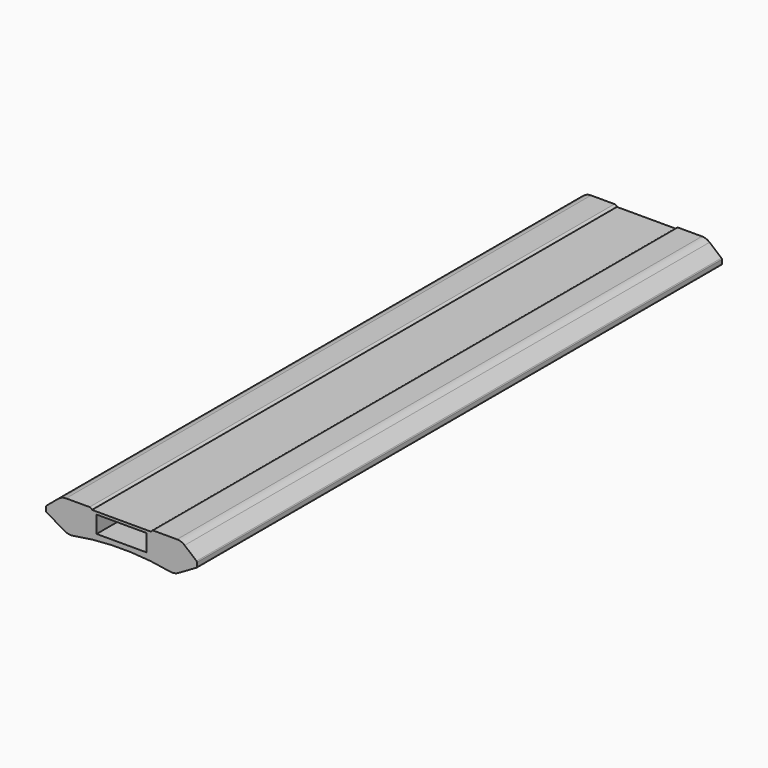
from build123d import *

# Parameters (mm, degrees)
F1_DEPTH    = 250
F2_W        = 38
F2_H        = 13
F3_DEPTH    = 250
F4_T1_DEPTH = 509.3674969976
F5_R        = 9
F6_R        = 1


# Not quite as in the source:
# - a fillet or chamfer that OpenCascade refuses, or shapes differently, is made with other operations: its cross-section is extruded or revolved along the edge and cut away or added


with BuildPart() as f1:
    # F0 (on Front) → F1 (new body, symmetric)
    with BuildSketch(Plane.XZ):
        with BuildLine():
            Line((22.5, 16.4041765079), (0, 16.4041765079))
            Line((0, 16.4041765079), (-22.5, 16.4041765079))
            Line((-22.5, 16.4041765079), (-22.5, 17.7041765079))
            Line((-22.5, 17.7041765079), (-45.5824640741, 17.7041765079))
            Line((-45.5824640741, 17.7041765079), (-57.5, 7.7041765079))
            Line((-57.5, 7.7041765079), (-57.5, 3.7041765079))
            Line((-57.5, 3.7041765079), (-40.1794919243, -6.2958234921))
            ThreePointArc((-40.1794919243, -6.2958234921), (0, -2.2182786337), (40.1794919243, -6.2958234921))
            Line((40.1794919243, -6.2958234921), (57.5, 3.7041765079))
            Line((57.5, 3.7041765079), (57.5, 7.7041765079))
            Line((57.5, 7.7041765079), (45.5824640741, 17.7041765079))
            Line((45.5824640741, 17.7041765079), (22.5, 17.7041765079))
            Line((22.5, 17.7041765079), (22.5, 16.4041765079))
        make_face()
    extrude(amount=F1_DEPTH, both=True)

    # F2 (on Front) → F3 (cut, symmetric)
    with BuildSketch(Plane.XZ):
        with Locations((0, 7.9041765079)):
            Rectangle(F2_W, F2_H)
    extrude(amount=F3_DEPTH, both=True, mode=Mode.SUBTRACT)

    # F4: fillet of radius 2 on 2 edges, made by hand

    # F4_s2 → F4_t1 (cut)
    with BuildSketch(Plane.XZ.offset(-254.6837484988)):
        with BuildLine():
            ThreePointArc((-22.5, 16.4041765079), (-23.2333239744, 17.3473441804), (-24.3734993995, 17.7041765079))
            Line((-24.3734993995, 17.7041765079), (-22.5, 17.7041765079))
            Line((-22.5, 17.7041765079), (-22.5, 16.4041765079))
        make_face()
        with BuildLine():
            ThreePointArc((24.3734993995, 17.7041765079), (23.2333239744, 17.3473441804), (22.5, 16.4041765079))
            Line((22.5, 16.4041765079), (22.5, 17.7041765079))
            Line((22.5, 17.7041765079), (24.3734993995, 17.7041765079))
        make_face()
    extrude(amount=F4_T1_DEPTH, mode=Mode.SUBTRACT)

    # F5
    f5_edges = [f1.edges().sort_by_distance(p)[0] for p in [
        (45.582464, 0, 17.704177),
        (40.179492, 0, -6.295823),
        (-40.179492, 0, -6.295823),
        (-45.582464, 0, 17.704177),
    ]]
    fillet(f5_edges, radius=F5_R)

    # F6
    f6_edges = [f1.edges().sort_by_distance(p)[0] for p in [
        (57.5, 0, 3.704177),
        (57.5, 0, 7.704177),
        (-57.5, 0, 7.704177),
        (-57.5, 0, 3.704177),
    ]]
    fillet(f6_edges, radius=F6_R)


solid = f1.part
